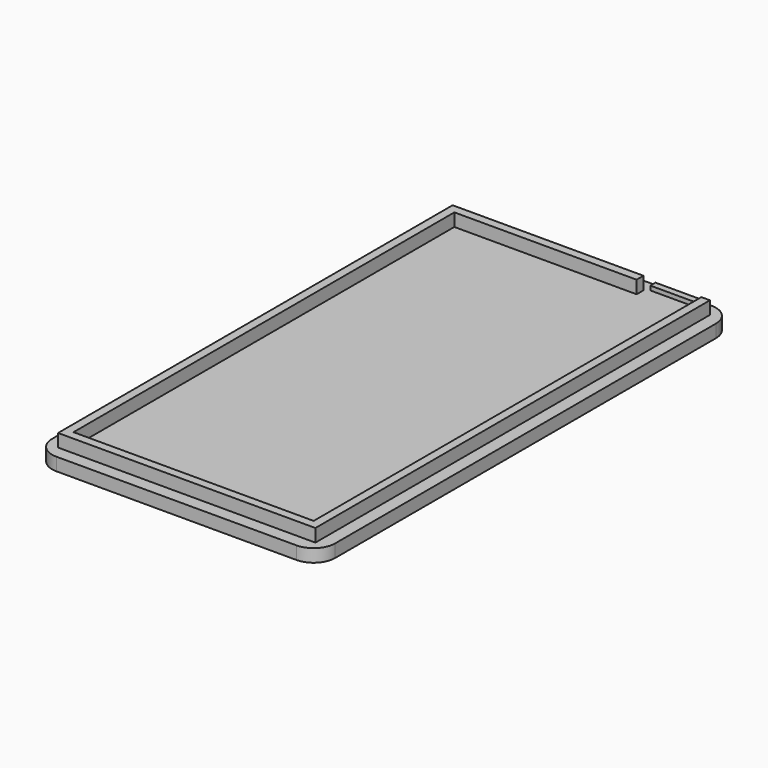
from build123d import *

# Parameters (mm, degrees)
F1_DEPTH = 6
F0_W     = 66
F0_H     = 121
F0_W_2   = 11.5
F0_H_2   = 1.5
F2_DEPTH = 3
F3_R     = 5
F4_DEPTH = 4


# Not quite as in the source:
# - a feature names something its author has since deleted; it is built from what else it names


with BuildPart() as f1:
    # F0 (on Top) → F1 (new body)
    with BuildSketch(Plane.XY):
        Polygon((30, -57.5), (30, 57.5), (28, 57.5), (28, -55.5), (-28, -55.5), (-28, 55.5), (14.5, 55.5), (14.5, 57.5), (-30, 57.5), (-30, -57.5), align=None)
    extrude(amount=F1_DEPTH)

    # F0 (on Top) → F2 (join)
    with BuildSketch(Plane.XY):
        Rectangle(F0_W, F0_H)
        Polygon((28, 57.5), (30, 57.5), (30, -57.5), (-30, -57.5), (-30, 57.5), (14.5, 57.5), (14.5, 55.5), (-28, 55.5), (-28, -55.5), (28, -55.5), align=None, mode=Mode.SUBTRACT)
        with Locations((21.25, 59)):
            Rectangle(F0_W_2, F0_H_2, mode=Mode.SUBTRACT)
    extrude(amount=F2_DEPTH)

    # F3
    f3_edges = [f1.edges().sort_by_distance(p)[0] for p in [
        (-33, 60.5, 1.5),
        (-33, -60.5, 1.5),
        (33, -60.5, 1.5),
        (33, 60.5, 1.5),
    ]]
    fillet(f3_edges, radius=F3_R)

    # F0 (on Top) → F4 (join)
    with BuildSketch(Plane.XY):
        with Locations((21.25, 59)):
            Rectangle(F0_W_2, F0_H_2)
    extrude(amount=F4_DEPTH)


solid = f1.part
